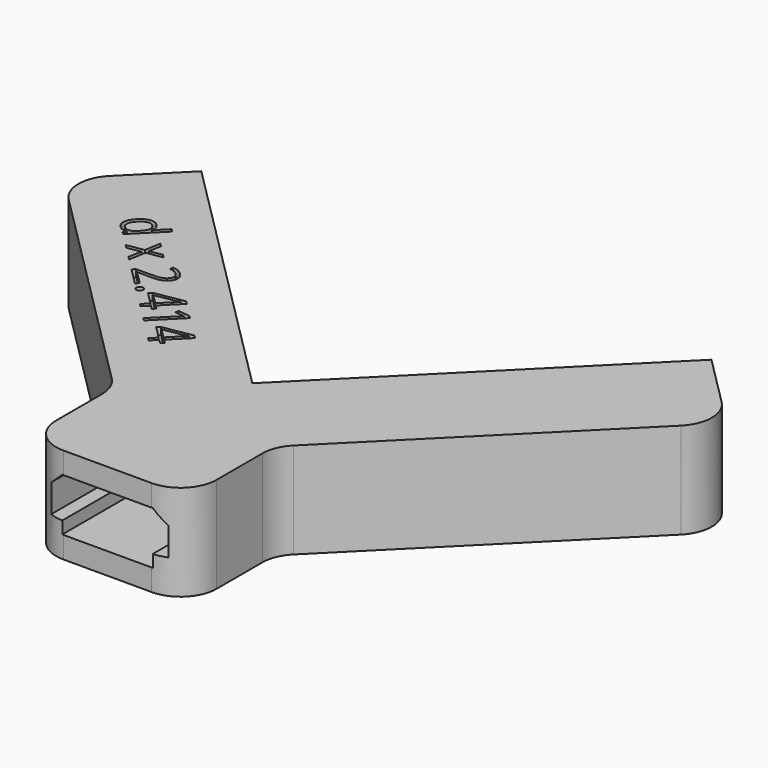
from build123d import *

# Parameters (mm, degrees)
F1_DEPTH     = 13.3
F2_W         = 12.55
F2_H         = 1.71
F2_H_2       = 5.59
F3_DEPTH     = 25.088
F4_W         = 4.05
F4_H         = 1.95
F5_DEPTH     = 35.3565424949
F6_TEXT_SIZE = 7.0518235575
F7_DEPTH     = 1


# Not quite as in the source:
# - Text() gives the source's letters only with a copy of the font that has no kerning and outlines rounded to 1/6400 em; it was checked with that copy


with BuildPart() as f1:
    # F0 (on Top) → F1 (new body)
    with BuildSketch(Plane.XY):
        with BuildLine():
            Line((35.3553390593, 35.3553390593), (0, 0))
            Line((0, 0), (-35.3553390593, 35.3553390593))
            Line((-35.3553390593, 35.3553390593), (-42.4264068712, 28.2842712475))
            ThreePointArc((-42.4264068712, 28.2842712475), (-43.8908729653, 24.7487373415), (-42.4264068712, 21.2132034356))
            Line((-42.4264068712, 21.2132034356), (-12.5894660941, -8.6237373415))
            ThreePointArc((-12.5894660941, -8.6237373415), (-11.5056023374, -10.2458540856), (-11.125, -12.1592712475))
            Line((-11.125, -12.1592712475), (-11.125, -20.0882034356))
            ThreePointArc((-11.125, -20.0882034356), (-9.6605339059, -23.6237373415), (-6.125, -25.0882034356))
            Line((-6.125, -25.0882034356), (6.125, -25.0882034356))
            ThreePointArc((6.125, -25.0882034356), (9.6605339059, -23.6237373415), (11.125, -20.0882034356))
            Line((11.125, -20.0882034356), (11.125, -12.1592712475))
            ThreePointArc((11.125, -12.1592712475), (11.5056023374, -10.2458540856), (12.5894660941, -8.6237373415))
            Line((12.5894660941, -8.6237373415), (42.4264068712, 21.2132034356))
            ThreePointArc((42.4264068712, 21.2132034356), (43.8908729653, 24.7487373415), (42.4264068712, 28.2842712475))
            Line((42.4264068712, 28.2842712475), (35.3553390593, 35.3553390593))
        make_face()
    extrude(amount=F1_DEPTH)

    # F2 (on face) → F3 (cut)
    with BuildSketch(Plane.XZ.offset(25.0882034356)):
        Polygon((6.275, 4.71), (8.125, 4.71), (8.125, 8.59), (6.275, 10.3), align=None)
        with Locations((0, 3.855)):
            Rectangle(F2_W, F2_H)
        with Locations((0, 7.505)):
            Rectangle(F2_W, F2_H_2)
        Polygon((-8.125, 4.71), (-6.275, 4.71), (-6.275, 10.3), (-8.125, 8.59), align=None)
    extrude(amount=-F3_DEPTH, mode=Mode.SUBTRACT)

    # F4 (on face) → F5 (cut, through all)
    with BuildSketch(Plane.XZ.offset(0.0002034356)):
        with Locations((0, 6.285)):
            Rectangle(F4_W, F4_H)
    extrude(amount=-F5_DEPTH, mode=Mode.SUBTRACT)

    # F6 (on face) → F7 (cut)
    with BuildSketch(Plane.XY.offset(13.3)):
        with Locations(Location((-35.3906943984, 21.1778480965), (0, 0, -45))):
            Text('d x 2.414', F6_TEXT_SIZE, font='Open Sans', text_align=(TextAlign.LEFT, TextAlign.BOTTOM))
    extrude(amount=-F7_DEPTH, mode=Mode.SUBTRACT)


solid = f1.part
